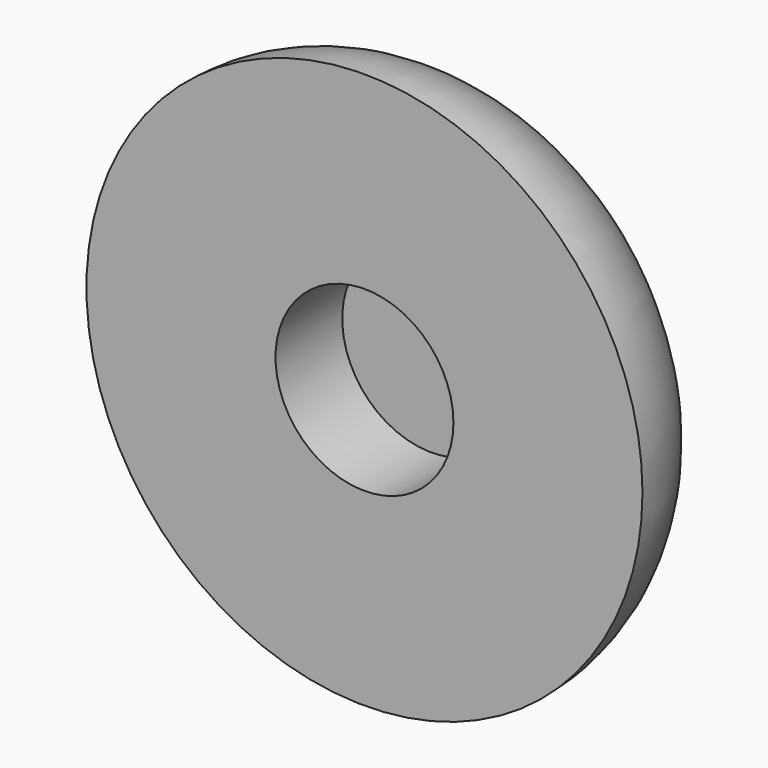
from build123d import *

# Parameters (mm, degrees)
F0_R     = 10
F1_DEPTH = 5
F2_R     = 4.99999
F3_R     = 3.2
F4_DEPTH = 3


# Not quite as in the source:
# - a fillet or chamfer is up to 0.001 mm smaller than in the source, because OpenCascade refuses the exact size


with BuildPart() as f1:
    # F0 (on Front) → F1 (new body)
    with BuildSketch(Plane.XZ):
        Circle(F0_R)
    extrude(amount=-F1_DEPTH)

    # F2 (radius 5 in the source; OpenCascade refuses exactly that, so slightly less here)
    f2_edges = [f1.edges().sort_by_distance(p)[0] for p in [
        (-10, 5, 0),
    ]]
    fillet(f2_edges, radius=F2_R)

    # F3 (on Front) → F4 (cut)
    with BuildSketch(Plane.XZ):
        Circle(F3_R)
    extrude(amount=-F4_DEPTH, mode=Mode.SUBTRACT)


solid = f1.part
